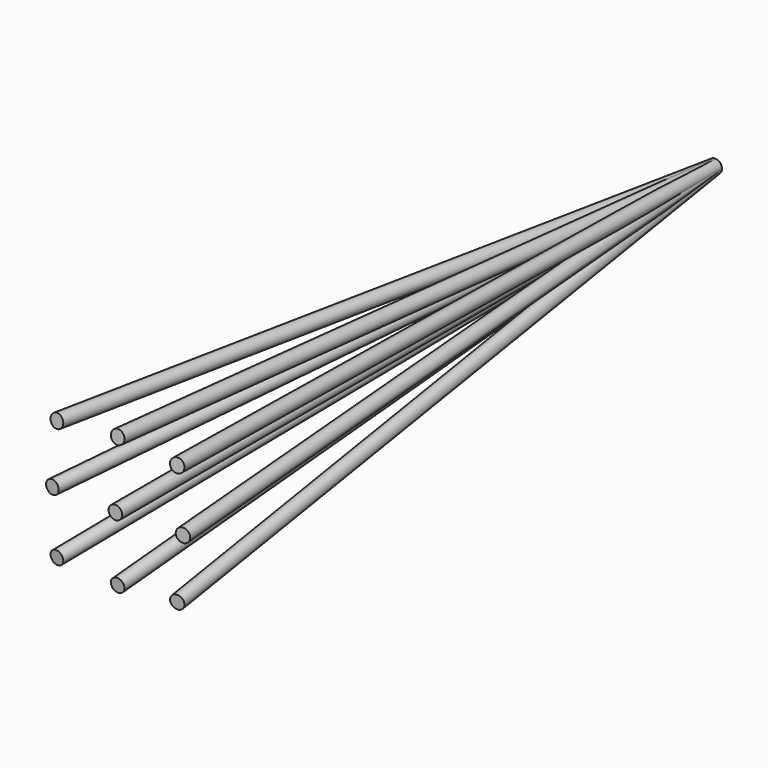
from build123d import *

# Parameters (mm, degrees)
F0_R      = 0.254
F1_DEPTH  = 27.94
F4_R      = 0.254
F5_DEPTH  = 27.94
F7_R      = 0.254
F8_DEPTH  = 27.94
F11_R     = 0.254
F12_DEPTH = 27.94
F14_R     = 0.254
F15_DEPTH = 27.94
F18_R     = 0.254
F19_DEPTH = 28.0416
F21_R     = 0.254
F22_DEPTH = 28.0416
F24_R     = 0.254
F25_DEPTH = 28.0416
F27_R     = 0.254
F28_DEPTH = 28.0416


with BuildPart() as f1:
    # F0 (on Front) → F1 (new body)
    with BuildSketch(Plane.XZ):
        Circle(F0_R)
    extrude(amount=F1_DEPTH)

    # F4 (on line) → F5 (join)
    with BuildSketch(Plane(origin=(0, 0, 0), x_dir=(-0.9961946981, 0.0871557427, 0), z_dir=(0.0871557427, 0.9961946981, 0))):
        Circle(F4_R)
    extrude(amount=-F5_DEPTH)

    # F7 (on line) → F8 (join)
    with BuildSketch(Plane(origin=(0, 0, 0), x_dir=(0.9961946981, 0.0871557427, 0), z_dir=(0.0871557427, -0.9961946981, 0))):
        Circle(F7_R)
    extrude(amount=F8_DEPTH)

    # F11 (on line) → F12 (join)
    with BuildSketch(Plane(origin=(0, 0, 0), x_dir=(-1, 0, 0), z_dir=(0, 0.9961946981, 0.0871557427))):
        Circle(F11_R)
    extrude(amount=-F12_DEPTH)

    # F14 (on line) → F15 (join)
    with BuildSketch(Plane(origin=(0, 0, 0), x_dir=(1, 0, 0), z_dir=(0, -0.9961946981, 0.0871557427))):
        Circle(F14_R)
    extrude(amount=F15_DEPTH)

    # F18 (on line) → F19 (join)
    with BuildSketch(Plane(origin=(0, 0, 0), x_dir=(-0.9967911096, -0.0797882397, -0.0064281109), z_dir=(-0.0800467601, 0.9935718557, 0.0800467601))):
        Circle(F18_R)
    extrude(amount=-F19_DEPTH)

    # F21 (on line) → F22 (join)
    with BuildSketch(Plane(origin=(0, 0, 0), x_dir=(0.9967911096, -0.0797882397, 0.0064281109), z_dir=(-0.0800467601, -0.9935718557, 0.0800467601))):
        Circle(F21_R)
    extrude(amount=F22_DEPTH)

    # F24 (on line) → F25 (join)
    with BuildSketch(Plane(origin=(0, 0, 0), x_dir=(-0.9967911096, -0.0797882397, 0.0064281109), z_dir=(-0.0800467601, 0.9935718557, -0.0800467601))):
        Circle(F24_R)
    extrude(amount=-F25_DEPTH)

    # F27 (on line) → F28 (join)
    with BuildSketch(Plane(origin=(0, 0, 0), x_dir=(0.9967911096, -0.0797882397, -0.0064281109), z_dir=(-0.0800467601, -0.9935718557, -0.0800467601))):
        Circle(F27_R)
    extrude(amount=F28_DEPTH)


solid = f1.part
